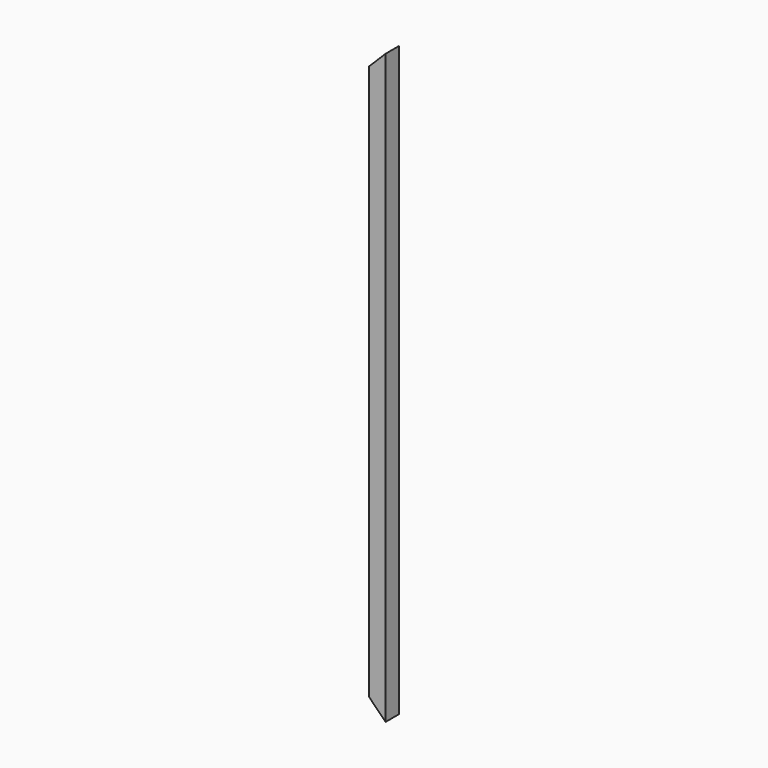
from build123d import *

# Parameters (mm, degrees)
F0_W        = 40
F0_H        = 40
F0_W_2      = 36
F0_H_2      = 36
F1_DEPTH    = 1430
F2_T1_DEPTH = 245.7346390373


# Not quite as in the source:
# - a fillet or chamfer that OpenCascade refuses, or shapes differently, is made with other operations: its cross-section is extruded or revolved along the edge and cut away or added


with BuildPart() as f1:
    # F0 (on Top) → F1 (new body)
    with BuildSketch(Plane.XY):
        with Locations((20, 20)):
            Rectangle(F0_W, F0_H)
        with Locations((20, 20)):
            Rectangle(F0_W_2, F0_H_2, mode=Mode.SUBTRACT)
    extrude(amount=F1_DEPTH)

    # F2: chamfer of 40 on 2 edges, made by hand

    # F2_s2 → F2_t1 (cut)
    with BuildSketch(Plane.XZ.offset(-142.8673195186)):
        Polygon((0, 40), (40, 0), (0, 0), align=None)
        Polygon((0, 1390), (40, 1430), (0, 1430), align=None)
    extrude(amount=F2_T1_DEPTH, mode=Mode.SUBTRACT)


solid = f1.part
